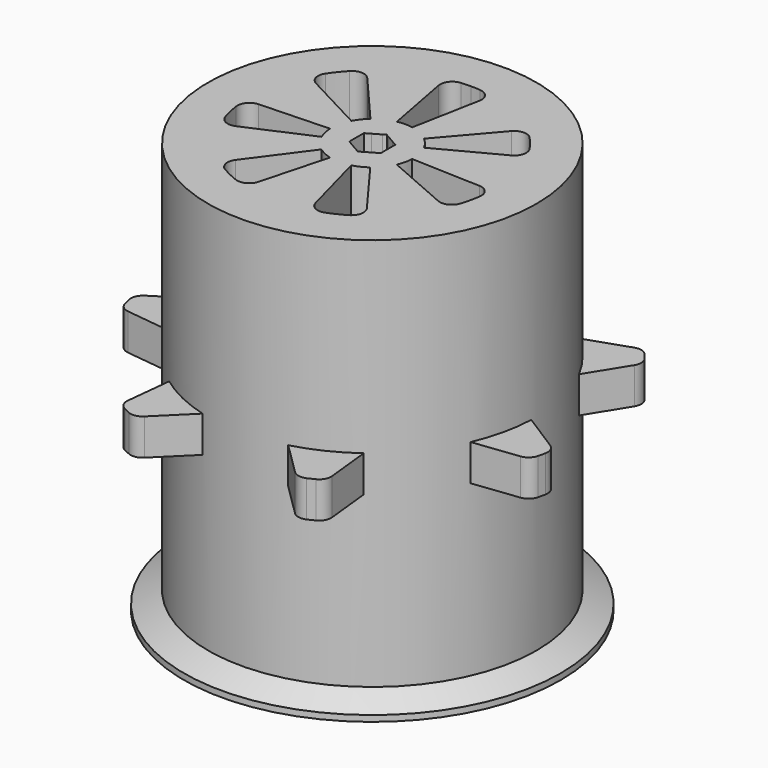
from build123d import *

# Parameters (mm, degrees)
F0_R     = 13.57391
F1_DEPTH = 17
F3_DEPTH = 1.5
F5_DEPTH = 34
F6_R     = 1
F7_R     = 15.57391
F7_R_2   = 13.57391
F8_DEPTH = 1.5
F9_SIZE2 = 0.99999
F9_SIZE  = 1.99999
F10_R    = 1


# Not quite as in the source:
# - a fillet or chamfer is up to 0.001 mm smaller than in the source, because OpenCascade refuses the exact size


with BuildPart() as f1:
    # F0 (on Top) → F1 (new body, symmetric)
    with BuildSketch(Plane.XY):
        Circle(F0_R)
    extrude(amount=F1_DEPTH, both=True)

    # F2 (on Top) → F3 (join, symmetric)
    with BuildSketch(Plane.XY):
        with BuildLine():
            Line((-8.8722387473, 10.27299432), (-13.094084175, 11.721231689))
            ThreePointArc((-13.094084175, 11.721231689), (-13.7398361081, 10.9571536638), (-14.3410637787, 10.1575687241))
            Line((-14.3410637787, 10.1575687241), (-11.9896877566, 6.3638369077))
            ThreePointArc((-11.9896877566, 6.3638369077), (-10.6125101782, 8.4631944563), (-8.8722387473, 10.27299432))
        make_face()
        with BuildLine():
            ThreePointArc((1, 17.5454356654), (0, 17.57391), (-1, 17.5454356654))
            Line((-1, 17.5454356654), (-2.5, 13.3417027657))
            ThreePointArc((-2.5, 13.3417027657), (0, 13.57391), (2.5, 13.3417027657))
            Line((2.5, 13.3417027657), (1, 17.5454356654))
        make_face()
        with BuildLine():
            Line((11.9896877566, 6.3638369077), (14.3410637787, 10.1575687241))
            ThreePointArc((14.3410637787, 10.1575687241), (13.7398361081, 10.9571536638), (13.094084175, 11.721231689))
            Line((13.094084175, 11.721231689), (8.8722387473, 10.27299432))
            ThreePointArc((8.8722387473, 10.27299432), (10.6125101782, 8.4631944563), (11.9896877566, 6.3638369077))
        make_face()
        with BuildLine():
            Line((12.4508960874, -5.4061279404), (16.8830140276, -4.8791546431))
            ThreePointArc((16.8830140276, -4.8791546431), (17.1332953852, -3.9105628665), (17.3280558955, -2.9292988187))
            Line((17.3280558955, -2.9292988187), (13.5635007572, -0.5314883795))
            ThreePointArc((13.5635007572, -0.5314883795), (13.2335837364, -3.0204791306), (12.4508960874, -5.4061279404))
        make_face()
        with BuildLine():
            Line((3.5363257124, -13.1051681845), (6.711710363, -16.2417750474))
            ThreePointArc((6.711710363, -16.2417750474), (7.6250337817, -15.8335457973), (8.5136480988, -15.3740075692))
            Line((8.5136480988, -15.3740075692), (8.0411700519, -10.9357494889))
            ThreePointArc((8.0411700519, -10.9357494889), (5.8894988252, -12.2296703257), (3.5363257124, -13.1051681845))
        make_face()
        with BuildLine():
            Line((-8.0411700519, -10.9357494889), (-8.5136480988, -15.3740075692))
            ThreePointArc((-8.5136480988, -15.3740075692), (-7.6250337817, -15.8335457973), (-6.711710363, -16.2417750474))
            Line((-6.711710363, -16.2417750474), (-3.5363257124, -13.1051681845))
            ThreePointArc((-3.5363257124, -13.1051681845), (-5.8894988252, -12.2296703257), (-8.0411700519, -10.9357494889))
        make_face()
        with BuildLine():
            Line((-13.5635007572, -0.5314883795), (-17.3280558955, -2.9292988187))
            ThreePointArc((-17.3280558955, -2.9292988187), (-17.1332953852, -3.9105628665), (-16.8830140276, -4.8791546431))
            Line((-16.8830140276, -4.8791546431), (-12.4508960874, -5.4061279404))
            ThreePointArc((-12.4508960874, -5.4061279404), (-13.2335837364, -3.0204791306), (-13.5635007572, -0.5314883795))
        make_face()
    extrude(amount=F3_DEPTH, both=True)

    # F4 (on face) → F5 (cut)
    with BuildSketch(Plane.XY.offset(17)):
        with BuildLine():
            ThreePointArc((-3.0007085232, 1.5847516846), (-2.6531275445, 2.1157986141), (-2.2127391143, 2.5728340707))
            Line((-2.2127391143, 2.5728340707), (-6.6382173429, 7.718502212))
            ThreePointArc((-6.6382173429, 7.718502212), (-7.9593826336, 6.3473958423), (-9.0021255696, 4.7542550537))
            Line((-9.0021255696, 4.7542550537), (-3.0007085232, 1.5847516846))
        make_face()
        with BuildLine():
            ThreePointArc((-0.6319024037, 3.334124907), (-0.3173418417, 3.3786067688), (0, 3.3934775))
            Line((0, 3.3934775), (0, 6.786955))
            Line((0, 6.786955), (0, 10.1804325))
            ThreePointArc((0, 10.1804325), (-0.9520255252, 10.1358203065), (-1.895707211, 10.0023747209))
            Line((-1.895707211, 10.0023747209), (-0.6319024037, 3.334124907))
        make_face()
        with BuildLine():
            Line((0, 6.786955), (0, 3.3934775))
            ThreePointArc((0, 3.3934775), (0.3173418417, 3.3786067688), (0.6319024037, 3.334124907))
            Line((0.6319024037, 3.334124907), (1.895707211, 10.0023747209))
            ThreePointArc((1.895707211, 10.0023747209), (0.9520255252, 10.1358203065), (0, 10.1804325))
            Line((0, 10.1804325), (0, 6.786955))
        make_face()
        with BuildLine():
            ThreePointArc((2.2127391143, 2.5728340707), (2.6531275445, 2.1157986141), (3.0007085232, 1.5847516846))
            Line((3.0007085232, 1.5847516846), (9.0021255696, 4.7542550537))
            ThreePointArc((9.0021255696, 4.7542550537), (7.9593826336, 6.3473958423), (6.6382173429, 7.718502212))
            Line((6.6382173429, 7.718502212), (2.2127391143, 2.5728340707))
        make_face()
        with BuildLine():
            ThreePointArc((3.3911429475, -0.1258532971), (3.3083959341, -0.7551197827), (3.1099199215, -1.3579718793))
            Line((3.1099199215, -1.3579718793), (9.3297597644, -4.073915638))
            ThreePointArc((9.3297597644, -4.073915638), (9.9251878023, -2.265359348), (10.1734288426, -0.3775598913))
            Line((10.1734288426, -0.3775598913), (3.3911429475, -0.1258532971))
        make_face()
        with BuildLine():
            ThreePointArc((2.0159469746, -2.7297705652), (1.4723747063, -3.0574175814), (0.8772981881, -3.2781149205))
            Line((0.8772981881, -3.2781149205), (2.6318945642, -9.8343447616))
            ThreePointArc((2.6318945642, -9.8343447616), (4.4171241189, -9.1722527443), (6.0478409237, -8.1893116956))
            Line((6.0478409237, -8.1893116956), (2.0159469746, -2.7297705652))
        make_face()
        with BuildLine():
            ThreePointArc((-0.8772981881, -3.2781149205), (-1.4723747063, -3.0574175814), (-2.0159469746, -2.7297705652))
            Line((-2.0159469746, -2.7297705652), (-6.0478409237, -8.1893116956))
            ThreePointArc((-6.0478409237, -8.1893116956), (-4.4171241189, -9.1722527443), (-2.6318945642, -9.8343447616))
            Line((-2.6318945642, -9.8343447616), (-0.8772981881, -3.2781149205))
        make_face()
        with BuildLine():
            ThreePointArc((-3.1099199215, -1.3579718793), (-3.3083959341, -0.7551197827), (-3.3911429475, -0.1258532971))
            Line((-3.3911429475, -0.1258532971), (-10.1734288426, -0.3775598913))
            ThreePointArc((-10.1734288426, -0.3775598913), (-9.9251878023, -2.265359348), (-9.3297597644, -4.073915638))
            Line((-9.3297597644, -4.073915638), (-3.1099199215, -1.3579718793))
        make_face()
        Polygon((-1.2990381057, 0.68605558), (0, 0), (-0.8620256343, 1.002309268), (-1.2990381057, 0.75), align=None)
        Polygon((-0.8620256343, 1.002309268), (0, 0), (-0.2562490973, 1.3520545147), align=None)
        Polygon((-0.2562490973, 1.3520545147), (0, 0), (0, 1.5), align=None)
        Polygon((0, 1.5), (0, 0), (0.2562490973, 1.3520545147), align=None)
        Polygon((0.2562490973, 1.3520545147), (0, 0), (0.8620256343, 1.002309268), align=None)
        Polygon((0.8620256343, 1.002309268), (0, 0), (1.2990381057, 0.68605558), (1.2990381057, 0.75), align=None)
        Polygon((1.2990381057, 0.68605558), (0, 0), (1.2990381057, -0.0482103619), align=None)
        Polygon((1.2990381057, -0.0482103619), (0, 0), (1.2990381057, -0.5672355759), align=None)
        Polygon((1.2990381057, -0.5672355759), (0, 0), (0.7766231283, -1.0516164278), (1.2990381057, -0.75), align=None)
        Polygon((0.7766231283, -1.0516164278), (0, 0), (0.3477089236, -1.2992501593), align=None)
        Polygon((0.3477089236, -1.2992501593), (0, 0), (-0.3477089236, -1.2992501593), (0, -1.5), align=None)
        Polygon((-0.3477089236, -1.2992501593), (0, 0), (-0.7766231283, -1.0516164278), align=None)
        Polygon((-0.7766231283, -1.0516164278), (0, 0), (-1.2990381057, -0.5672355759), (-1.2990381057, -0.75), align=None)
        Polygon((-1.2990381057, -0.5672355759), (0, 0), (-1.2990381057, -0.0482103619), align=None)
        Polygon((-1.2990381057, -0.0482103619), (0, 0), (-1.2990381057, 0.68605558), align=None)
    extrude(amount=-F5_DEPTH, mode=Mode.SUBTRACT)

    # F6
    f6_edges = [f1.edges().sort_by_distance(p)[0] for p in [
        (-6.047841, -8.189312, 0),
        (-2.631895, -9.834345, 0),
        (2.631895, -9.834345, 0),
        (6.047841, -8.189312, 0),
        (9.32976, -4.073916, 0),
        (-9.32976, -4.073916, 0),
        (-10.173429, -0.37756, 0),
        (-9.002126, 4.754255, 0),
        (-6.638217, 7.718502, 0),
        (6.638217, 7.718502, 0),
        (-1.895707, 10.002375, 0),
        (1.895707, 10.002375, 0),
        (9.002126, 4.754255, 0),
        (10.173429, -0.37756, 0),
    ]]
    fillet(f6_edges, radius=F6_R)

    # F7 (on face) → F8 (join)
    with BuildSketch(Plane(origin=(0, 0, -17), x_dir=(1, 0, 0), z_dir=(0, 0, -1))):
        Circle(F7_R)
        Circle(F7_R_2, mode=Mode.SUBTRACT)
    extrude(amount=-F8_DEPTH)

    # F9 (size 2 and 1 in the source; OpenCascade refuses exactly that, so slightly less here)
    f9_edges = [f1.edges().sort_by_distance(p)[0] for p in [
        (-15.57391, 0, -15.5),
    ]]
    f9_side = f1.faces().sort_by_distance((-15.133413, 0, -15.5))[0]
    chamfer(f9_edges, length=F9_SIZE, length2=F9_SIZE2, reference=f9_side)

    # F10
    f10_edges = [f1.edges().sort_by_distance(p)[0] for p in [
        (14.341064, 10.157569, 0),
        (13.094084, 11.721232, 0),
        (1, 17.545436, 0),
        (-1, 17.545436, 0),
        (-13.094084, 11.721232, 0),
        (-14.341064, 10.157569, 0),
        (-17.328056, -2.929299, 0),
        (-16.883014, -4.879155, 0),
        (-8.513648, -15.374008, 0),
        (-6.71171, -16.241775, 0),
        (6.71171, -16.241775, 0),
        (8.513648, -15.374008, 0),
        (16.883014, -4.879155, 0),
        (17.328056, -2.929299, 0),
    ]]
    fillet(f10_edges, radius=F10_R)


solid = f1.part
